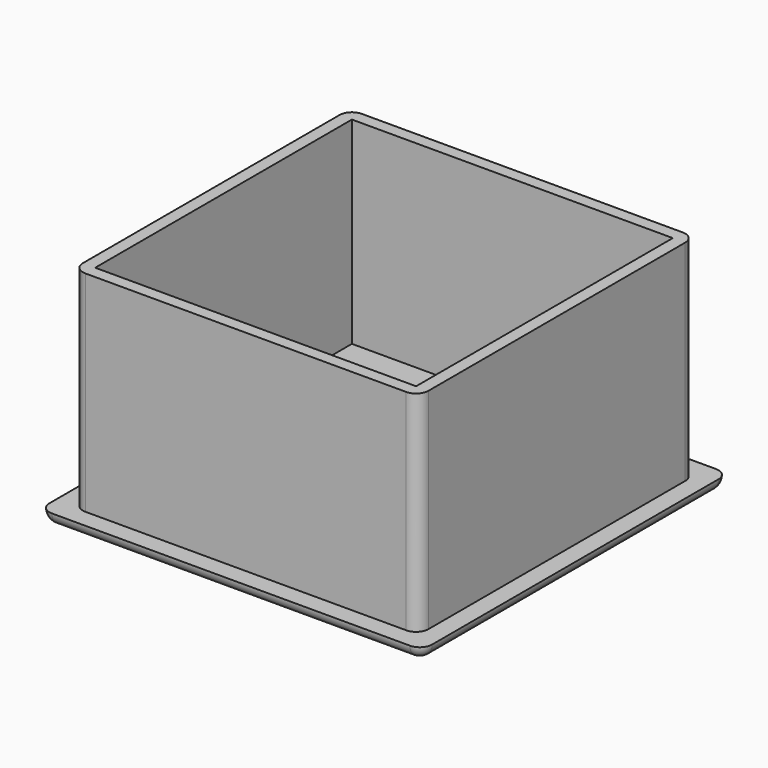
from build123d import *

# Parameters (mm, degrees)
F0_W     = 71.12
F0_H     = 71.12
F1_DEPTH = 43.18
F2_W     = 66.04
F2_H     = 66.04
F3_DEPTH = 40.64
F5_R     = 2.54
F4_W     = 71.12
F4_H     = 71.12
F4_W_2   = 3.81
F4_H_2   = 3.81
F6_DEPTH = 2.54
F7_R     = 2.53999


# Not quite as in the source:
# - a fillet or chamfer is up to 0.001 mm smaller than in the source, because OpenCascade refuses the exact size


with BuildPart() as f1:
    # F0 (on Top) → F1 (new body)
    with BuildSketch(Plane.XY):
        with Locations((35.56, 35.56)):
            Rectangle(F0_W, F0_H)
    extrude(amount=F1_DEPTH)

    # F2 (on face) → F3 (cut)
    with BuildSketch(Plane.XY.offset(43.18)):
        with Locations((35.56, 35.56)):
            Rectangle(F2_W, F2_H)
    extrude(amount=-F3_DEPTH, mode=Mode.SUBTRACT)

    # F5
    f5_edges = [f1.edges().sort_by_distance(p)[0] for p in [
        (71.12, 0, 21.59),
        (0, 0, 21.59),
        (0, 71.12, 21.59),
        (71.12, 71.12, 21.59),
    ]]
    fillet(f5_edges, radius=F5_R)

    # F4 (on face) → F6 (join)
    with BuildSketch(Plane(origin=(0, 0, 0), x_dir=(1, 0, 0), z_dir=(0, 0, -1))):
        Polygon((-3.81, -71.12), (0, -71.12), (0, -74.93), (74.93, -74.93), (74.93, 3.81), (-3.81, 3.81), align=None)
        with Locations((35.56, -35.56)):
            Rectangle(F4_W, F4_H, mode=Mode.SUBTRACT)
        with Locations((-1.905, -73.025)):
            Rectangle(F4_W_2, F4_H_2)
        with Locations((35.56, -35.56)):
            Rectangle(F4_W, F4_H)
    extrude(amount=F6_DEPTH)

    # F7 (radius 2.54 in the source; OpenCascade refuses exactly that, so slightly less here)
    f7_edges = [f1.edges().sort_by_distance(p)[0] for p in [
        (74.93, 35.56, -2.54),
        (35.56, -3.81, -2.54),
        (-3.81, 35.56, -2.54),
        (35.56, 74.93, -2.54),
        (-3.81, 74.93, -1.27),
        (74.93, 74.93, -1.27),
        (74.93, -3.81, -1.27),
        (-3.81, -3.81, -1.27),
    ]]
    fillet(f7_edges, radius=F7_R)


solid = f1.part
